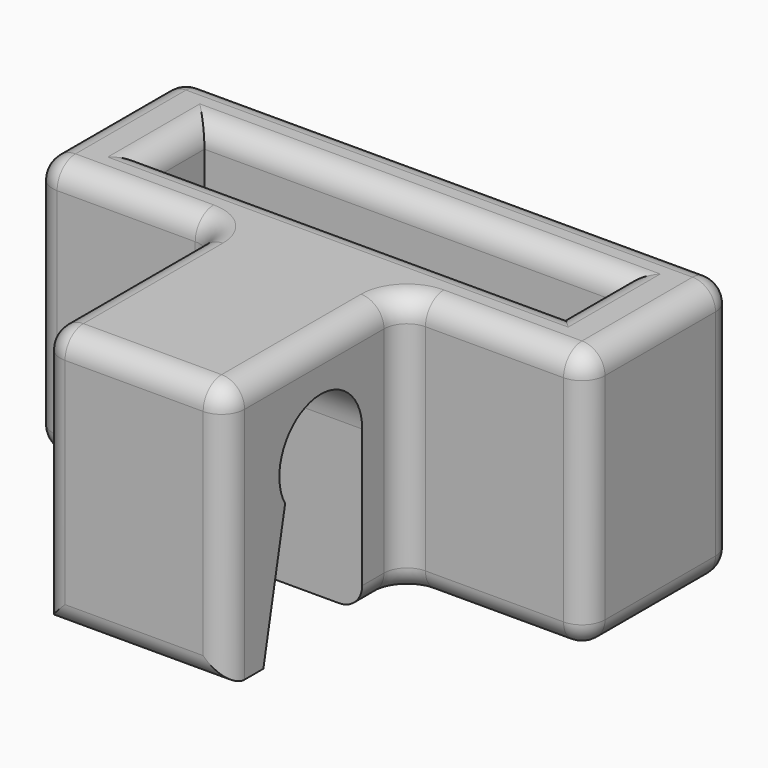
from build123d import *

# Parameters (mm, degrees)
F1_DEPTH = 8
F2_W     = 24
F2_H     = 11.337432079
F3_DEPTH = 8
F4_W     = 18
F4_H     = 3
F5_DEPTH = 11.338432079
F6_F1_R  = 1
F6_F2_R  = 1
F7_R     = 1.49999


# Not quite as in the source:
# - a fillet or chamfer is up to 0.001 mm smaller than in the source, because OpenCascade refuses the exact size


with BuildPart() as f1:
    # F0 (on Right) → F1 (new body)
    with BuildSketch(Plane.YZ):
        with BuildLine():
            ThreePointArc((-20.601621214, 10.7601184938), (-19.2613938683, 14.0777191086), (-16.4163531623, 11.9078281993))
            Line((-16.4163531623, 11.9078281993), (-16.4163531623, 4.9222996458))
            Line((-16.4163531623, 4.9222996458), (-14.2332110554, 4.9222996458))
            Line((-14.2332110554, 4.9222996458), (-14.2332110554, 16.2597317249))
            Line((-14.2332110554, 16.2597317249), (-23.8023772836, 16.2597317249))
            Line((-23.8023772836, 16.2597317249), (-23.8023772836, 4.9222996458))
            Line((-23.8023772836, 4.9222996458), (-21.7834785581, 4.9222996458))
            Line((-21.7834785581, 4.9222996458), (-20.601621214, 10.7601184938))
        make_face()
    extrude(amount=F1_DEPTH)

    # F2 (on face) → F3 (join)
    with BuildSketch(Plane(origin=(0, -14.2332110554, 0), x_dir=(-1, 0, 0), z_dir=(0, 1, 0))):
        with Locations((-4, 10.5910156853)):
            Rectangle(F2_W, F2_H)
    extrude(amount=F3_DEPTH)

    # F4 (on face) → F5 (cut, through all)
    with BuildSketch(Plane.XY.offset(16.2597317249)):
        with Locations((4, -10.2332110554)):
            Rectangle(F4_W, F4_H)
    extrude(amount=-F5_DEPTH, mode=Mode.SUBTRACT)

    # F6: fillet of radius 1 on 26 edges, made by hand

    # F6_f1
    f6_f1_edges = [f1.edges().sort_by_distance(p)[0] for p in [
        (0, -14.2332110554, 10.5910156853),
        (8, -14.2332110554, 10.5910156853),
    ]]
    fillet(f6_f1_edges, radius=F6_F1_R)

    # F6_f2
    f6_f2_edges = [f1.edges().sort_by_distance(p)[0] for p in [
        (-8, -10.2332110554, 16.2597317249),
        (-4.5, -14.2332110554, 16.2597317249),
        (4, -6.2332110554, 16.2597317249),
        (0, -19.5177941695, 16.2597317249),
        (16, -10.2332110554, 16.2597317249),
        (4, -23.8023772836, 16.2597317249),
        (12.5, -14.2332110554, 16.2597317249),
        (8, -19.5177941695, 16.2597317249),
        (-5, -10.2332110554, 16.2597317249),
        (4, -8.7332110554, 16.2597317249),
        (13, -10.2332110554, 16.2597317249),
        (4, -11.7332110554, 16.2597317249),
        (16, -10.2332110554, 4.9222996458),
        (16, -14.2332110554, 10.5910156853),
        (16, -6.2332110554, 10.5910156853),
        (4, -6.2332110554, 4.9222996458),
        (-8, -6.2332110554, 10.5910156853),
        (-8, -10.2332110554, 4.9222996458),
        (-8, -14.2332110554, 10.5910156853),
        (-4.5, -14.2332110554, 4.9222996458),
        (12.5, -14.2332110554, 4.9222996458),
        (4, -23.8023772836, 4.9222996458),
        (0, -23.8023772836, 10.5910156853),
        (8, -23.8023772836, 10.5910156853),
        (8.2928932188, -14.5261042742, 4.9222996458),
        (-0.2928932188, -14.5261042742, 4.9222996458),
        (8.2928932188, -14.5261042742, 16.2597317249),
        (-0.2928932188, -14.5261042742, 16.2597317249),
    ]]
    fillet(f6_f2_edges, radius=F6_F2_R)

    # F7 (radius 1.5 in the source; OpenCascade refuses exactly that, so slightly less here)
    f7_edges = [f1.edges().sort_by_distance(p)[0] for p in [
        (-5, -10.233211, 4.9223),
        (4, -11.733211, 4.9223),
        (4, -8.733211, 4.9223),
        (13, -10.233211, 4.9223),
    ]]
    fillet(f7_edges, radius=F7_R)


solid = f1.part
